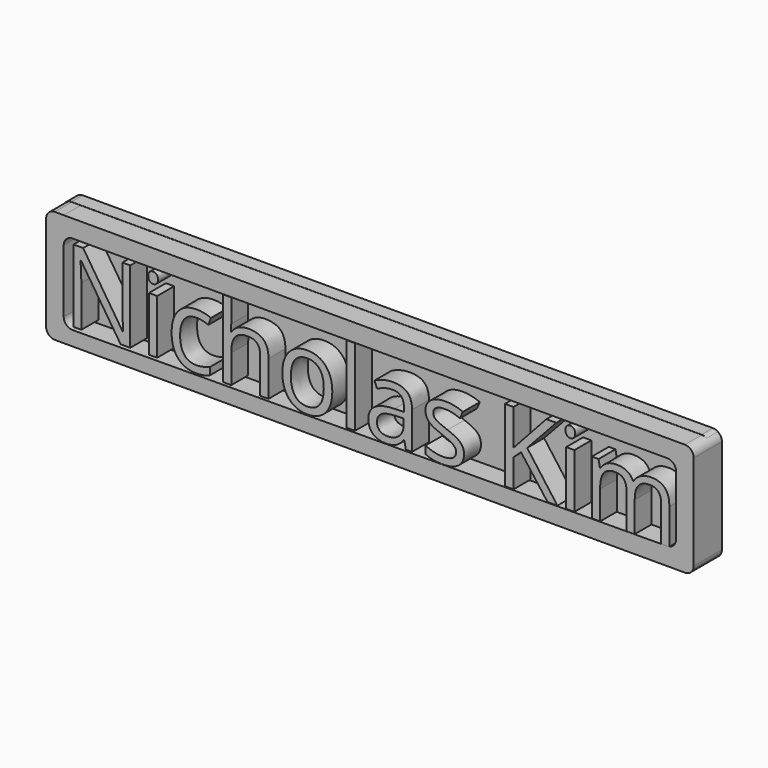
from build123d import *

# Parameters (mm, degrees)
F0_TEXT_SIZE = 73.1499568145
F2_DEPTH     = 25.4
F4_DEPTH     = 10.16
F5_DEPTH     = 25.4


# Not quite as in the source:
# - Text() gives the source's letters only with a copy of the font that has no kerning and outlines rounded to 1/6400 em; it was checked with that copy


with BuildPart() as f2:
    # F0 (on Front) → F2 (new body)
    with BuildSketch(Plane.XZ):
        with Locations((-220.5779254436, -15.565643087)):
            Text('Nicholas Kim', F0_TEXT_SIZE, font='Open Sans', text_align=(TextAlign.LEFT, TextAlign.BOTTOM))
    extrude(amount=F2_DEPTH)

    # F3 (on Front) → F4 (join)
    with BuildSketch(Plane.XZ):
        with BuildLine():
            Line((-227.0487653255, -28.1715746969), (226.5393393278, -28.1715746969))
            ThreePointArc((226.5393393278, -28.1715746969), (231.0294673883, -26.3117027574), (232.8893393278, -21.8215746969))
            Line((232.8893393278, -21.8215746969), (232.8893393278, 46.6902734876))
            ThreePointArc((232.8893393278, 46.6902734876), (231.0294673883, 51.1804015481), (226.5393393278, 53.0402734876))
            Line((226.5393393278, 53.0402734876), (-227.0487653255, 53.0402734876))
            ThreePointArc((-227.0487653255, 53.0402734876), (-231.5388933861, 51.1804015481), (-233.3987653255, 46.6902734876))
            Line((-233.3987653255, 46.6902734876), (-233.3987653255, -21.8215746969))
            ThreePointArc((-233.3987653255, -21.8215746969), (-231.5388933861, -26.3117027574), (-227.0487653255, -28.1715746969))
        make_face()
    extrude(amount=F4_DEPTH)


with BuildPart() as f5:
    # F1 (on Front) → F5 (new body)
    with BuildSketch(Plane.XZ):
        with BuildLine():
            Line((226.7336293483, 52.9193078749), (-220.5044776201, 52.9193181217))
            Line((-220.5044776201, 52.9193181217), (-226.8544776201, 52.9193181217))
            ThreePointArc((-226.8544776201, 52.9193181217), (-231.3446056807, 51.0594461822), (-233.2044776201, 46.5693181217))
            Line((-233.2044776201, 46.5693181217), (-233.2044776201, 40.2193181217))
            Line((-233.2044776201, 40.2193181217), (-233.2044776201, -21.8632198706))
            ThreePointArc((-233.2044776201, -21.8632198706), (-231.3446056807, -26.3533479312), (-226.8544776201, -28.2132198706))
            Line((-226.8544776201, -28.2132198706), (220.3836292028, -28.2132198706))
            Line((220.3836292028, -28.2132198706), (226.7336292028, -28.2132198706))
            ThreePointArc((226.7336292028, -28.2132198706), (231.2237572634, -26.3533479312), (233.0836292028, -21.8632198706))
            Line((233.0836292028, -21.8632198706), (233.0836292028, -15.5132198706))
            Line((233.0836292028, -15.5132198706), (233.0836292028, 46.5693078749))
            ThreePointArc((233.0836292028, 46.5693078749), (231.2237573148, 51.059435884), (226.7336293483, 52.9193078749))
        make_face()
        with BuildLine():
            Line((-220.5044776201, -11.4786624907), (-220.5044776201, 33.8693181217))
            ThreePointArc((-220.5044776201, 33.8693181217), (-218.6446056807, 38.3594461822), (-214.1544776201, 40.2193181217))
            Line((-214.1544776201, 40.2193181217), (214.0336292028, 40.2193181217))
            ThreePointArc((214.0336292028, 40.2193181217), (218.5237572634, 38.3594461822), (220.3836292028, 33.8693181217))
            Line((220.3836292028, 33.8693181217), (220.3836292028, -9.196967101))
            ThreePointArc((220.3836292028, -9.196967101), (218.5357045211, -13.6751160298), (214.0674661072, -15.5468769479))
            Line((214.0674661072, -15.5468769479), (-214.1206407158, -17.8285723376))
            ThreePointArc((-214.1206407158, -17.8285723376), (-218.6326265489, -15.980737809), (-220.5044776201, -11.4786624907))
        make_face(mode=Mode.SUBTRACT)
    extrude(amount=F5_DEPTH)


solid = Compound([f2.part, f5.part])
